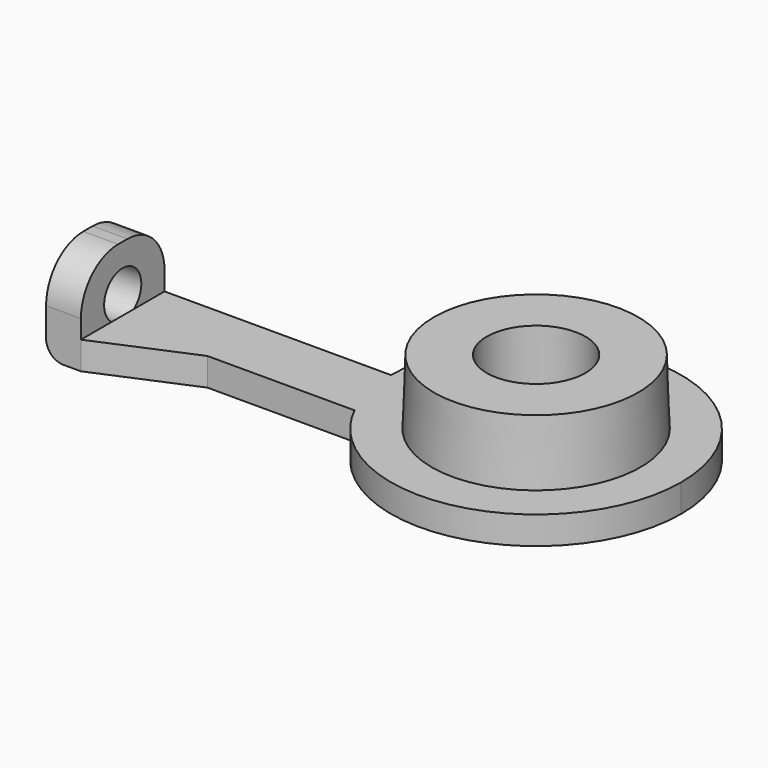
from build123d import *

# Parameters (mm, degrees)
F1_DEPTH    = 2.4
F0_W        = 3
F0_H        = 9
F2_DEPTH    = 8
F4_R        = 2
F5_DEPTH    = 3
F6_R        = 4
F7_T1_DEPTH = 16.5


# Not quite as in the source:
# - a fillet or chamfer that OpenCascade refuses, or shapes differently, is made with other operations: its cross-section is extruded or revolved along the edge and cut away or added


with BuildPart() as f1:
    # F0 (on Top) → F1 (new body)
    with BuildSketch(Plane.XY):
        with BuildLine():
            ThreePointArc((-9, 0), (-8.5094701622, -2.9306855101), (-7.0913516535, -5.5419068674))
            Line((-7.0913516535, -5.5419068674), (-4.1106286956, -5.5419068674))
            ThreePointArc((-4.1106286956, -5.5419068674), (-6.1633326212, -3.1021494161), (-6.9, 0))
            Line((-6.9, 0), (-9, 0))
        make_face()
        with BuildLine():
            ThreePointArc((-7.0913516535, -5.5419068674), (-3.9447964582, -8.0894116537), (0, -9))
            ThreePointArc((0, -9), (6.3639610307, -6.3639610307), (9, 0))
            ThreePointArc((9, 0), (0, 9), (-9, 0))
            Line((-9, 0), (-6.9, 0))
            ThreePointArc((-6.9, 0), (0, 6.9), (6.9, 0))
            ThreePointArc((6.9, 0), (3.1021494161, -6.1633326212), (-4.1106286956, -5.5419068674))
            Line((-4.1106286956, -5.5419068674), (-7.0913516535, -5.5419068674))
        make_face()
        with BuildLine():
            Line((-23.8745937477, -5.5419068674), (-11.2043414922, -5.5419068674))
            ThreePointArc((-11.2043414922, -5.5419068674), (-12.1717761369, -2.8456749066), (-12.5, 0))
            Line((-12.5, 0), (-32, 0))
            Line((-32, 0), (-32, -9))
            Line((-32, -9), (-23.8745937477, -5.5419068674))
        make_face()
        with BuildLine():
            ThreePointArc((9, 0), (6.3639610307, -6.3639610307), (0, -9))
            Line((0, -9), (-8.6746757864, -9))
            ThreePointArc((-8.6746757864, -9), (4.8896090165, -11.5039872942), (12.5, 0))
            ThreePointArc((12.5, 0), (0, 12.5), (-12.5, 0))
            Line((-12.5, 0), (-9, 0))
            ThreePointArc((-9, 0), (0, 9), (9, 0))
        make_face()
        with BuildLine():
            Line((-11.2043414922, -5.5419068674), (-7.0913516535, -5.5419068674))
            ThreePointArc((-7.0913516535, -5.5419068674), (-8.5094701622, -2.9306855101), (-9, 0))
            Line((-9, 0), (-12.5, 0))
            ThreePointArc((-12.5, 0), (-12.1717761369, -2.8456749066), (-11.2043414922, -5.5419068674))
        make_face()
        with BuildLine():
            Line((-8.6746757864, -9), (0, -9))
            ThreePointArc((0, -9), (-3.9447964582, -8.0894116537), (-7.0913516535, -5.5419068674))
            Line((-7.0913516535, -5.5419068674), (-11.2043414922, -5.5419068674))
            ThreePointArc((-11.2043414922, -5.5419068674), (-10.0887776276, -7.3801467452), (-8.6746757864, -9))
        make_face()
    extrude(amount=F1_DEPTH)

    # F0 (on Top) → F2 (join)
    with BuildSketch(Plane.XY):
        with BuildLine():
            ThreePointArc((-6.9, 0), (-6.1633326212, -3.1021494161), (-4.1106286956, -5.5419068674))
            ThreePointArc((-4.1106286956, -5.5419068674), (3.1021494161, -6.1633326212), (6.9, 0))
            ThreePointArc((6.9, 0), (0, 6.9), (-6.9, 0))
        make_face()
        with BuildLine():
            ThreePointArc((4.25, 0), (0, -4.25), (-4.25, 0))
            ThreePointArc((-4.25, 0), (0, 4.25), (4.25, 0))
        make_face(mode=Mode.SUBTRACT)
        with Locations((-33.5, -4.5)):
            Rectangle(F0_W, F0_H)
        with BuildLine():
            ThreePointArc((-7.0913516535, -5.5419068674), (-3.9447964582, -8.0894116537), (0, -9))
            ThreePointArc((0, -9), (6.3639610307, -6.3639610307), (9, 0))
            ThreePointArc((9, 0), (0, 9), (-9, 0))
            Line((-9, 0), (-6.9, 0))
            ThreePointArc((-6.9, 0), (0, 6.9), (6.9, 0))
            ThreePointArc((6.9, 0), (3.1021494161, -6.1633326212), (-4.1106286956, -5.5419068674))
            Line((-4.1106286956, -5.5419068674), (-7.0913516535, -5.5419068674))
        make_face()
        with BuildLine():
            ThreePointArc((-9, 0), (-8.5094701622, -2.9306855101), (-7.0913516535, -5.5419068674))
            Line((-7.0913516535, -5.5419068674), (-4.1106286956, -5.5419068674))
            ThreePointArc((-4.1106286956, -5.5419068674), (-6.1633326212, -3.1021494161), (-6.9, 0))
            Line((-6.9, 0), (-9, 0))
        make_face()
    extrude(amount=F2_DEPTH)

    # F4 (on offset) → F5 (cut, through all)
    with BuildSketch(Plane(origin=(-35, 0, 0), x_dir=(0, -1, 0), z_dir=(-1, 0, 0))):
        with Locations((4.5, 4)):
            Circle(F4_R)
    extrude(amount=-F5_DEPTH, mode=Mode.SUBTRACT)

    # F6
    f6_edges = [f1.edges().sort_by_distance(p)[0] for p in [
        (-33.5, -9, 8),
        (-33.5, 0, 8),
    ]]
    fillet(f6_edges, radius=F6_R)

    # F7: fillet of radius 1.5 on 2 edges, made by hand

    # F7_s2 → F7_t1 (cut)
    with BuildSketch(Plane.XZ.offset(-3.75)):
        with BuildLine():
            ThreePointArc((-35, 1.5), (-34.5606601718, 0.4393398282), (-33.5, 0))
            Line((-33.5, 0), (-35, 0))
            Line((-35, 0), (-35, 1.5))
        make_face()
    extrude(amount=F7_T1_DEPTH, mode=Mode.SUBTRACT)

    # F8: chamfer of 0.2 x 5.7272506566 on 1 edges, made by hand


with BuildPart() as f8_tool2:
    # F8_s3 → F8_t4 (revolve)
    with BuildSketch(Plane.XZ):
        Polygon((-9, 2.2727493434), (-8.8, 8), (-9, 8), align=None)
    revolve(axis=Axis((0, 0, 8), (0, 0, 1)))

    split(bisect_by=Plane.XY.offset(2.4), keep=Keep.TOP)


with BuildPart() as f1_1:
    add(f1.part)

    # F8_t1: cut F8_tool2
    add(f8_tool2.part, mode=Mode.SUBTRACT)


solid = f1_1.part
